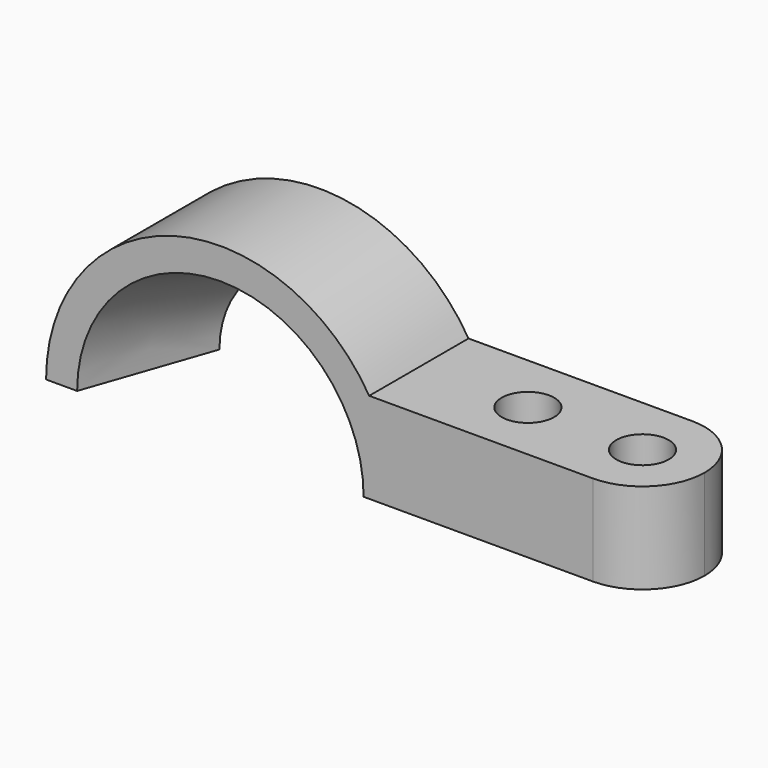
from build123d import *

# Parameters (mm, degrees)
F1_DEPTH = 52
F4_R     = 25.99999
F5_R     = 11
F6_DEPTH = 92


# Not quite as in the source:
# - a fillet or chamfer is up to 0.001 mm smaller than in the source, because OpenCascade refuses the exact size


with BuildPart() as f1:
    # F0 (on Front) → F1 (new body)
    with BuildSketch(Plane.XZ):
        with BuildLine():
            Line((182, 38), (62.329768169, 38))
            ThreePointArc((62.329768169, 38), (-19.7348286497, 70.2818364741), (-73, 0))
            Line((-73, 0), (182, 0))
            Line((182, 0), (182, 38))
        make_face()
    extrude(amount=F1_DEPTH)

    # F2 (on face) → F3 (revolve, cut)
    with BuildSketch(Plane(origin=(0, 0, 0), x_dir=(1, 0, 0), z_dir=(0, 0, -1))):
        Polygon((60, 52), (0, 52), (0, 0), (42, 0), align=None)
    revolve(axis=Axis((0, -26, 0), (0, 1, 0)), mode=Mode.SUBTRACT)

    # F4 (radius 26 in the source; OpenCascade refuses exactly that, so slightly less here)
    f4_edges = [f1.edges().sort_by_distance(p)[0] for p in [
        (182, -52, 19),
        (182, 0, 19),
    ]]
    fillet(f4_edges, radius=F4_R)

    # F5 (on face) → F6 (cut)
    with BuildSketch(Plane(origin=(0, 0, 0), x_dir=(1, 0, 0), z_dir=(0, 0, -1))):
        with Locations((108, 26)):
            Circle(F5_R)
        with Locations((156, 26)):
            Circle(F5_R)
    extrude(amount=-F6_DEPTH, mode=Mode.SUBTRACT)


solid = f1.part
